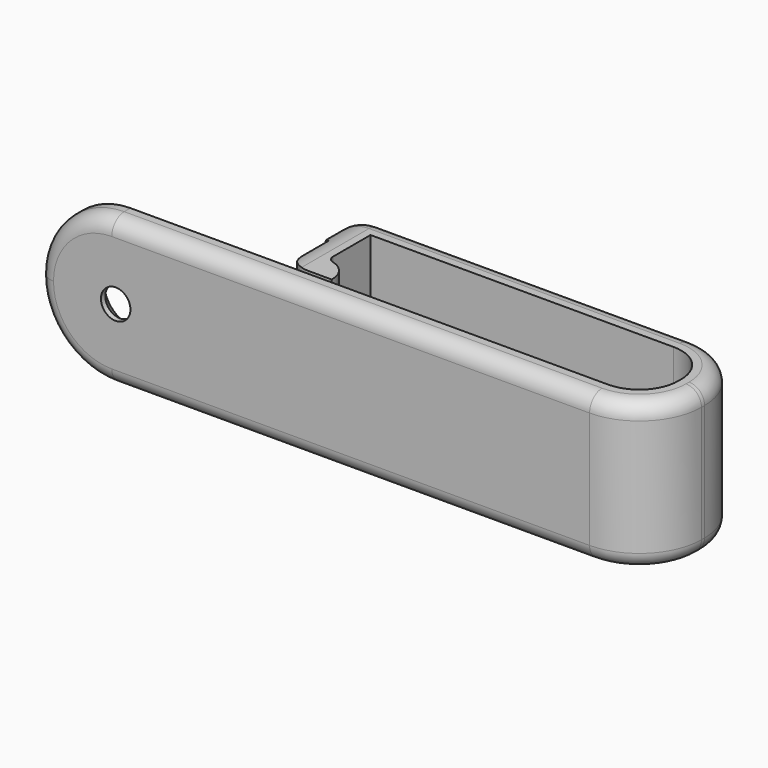
from build123d import *

# Parameters (mm, degrees)
F2_W            = 3
F2_H            = 3
F3_DEPTH        = 19
F5_R            = 9.49999
F6_R            = 5
F7_R            = 2
F8_R            = 1
F9_SIZE         = 2.99999
F10_D           = 3.7973
F10_CSINK_D     = 7.7978
F10_CSINK_ANGLE = 82
F11_R           = 2.9999


# Not quite as in the source:
# - a fillet or chamfer is up to 0.001 mm smaller than in the source, because OpenCascade refuses the exact size


with BuildPart() as f3:
    # F2 (on Top) → F3 (new body)
    with BuildSketch(Plane.XY):
        with BuildLine():
            Line((35.5, -27.8585158202), (-35.5, -27.8585158202))
            Line((-35.5, -27.8585158202), (-35.5, -30.8585158202))
            Line((-35.5, -30.8585158202), (35.5, -30.8585158202))
            ThreePointArc((35.5, -30.8585158202), (41.1568542495, -28.5153700696), (43.5, -22.8585158202))
            Line((43.5, -22.8585158202), (43.5, -22.3585158202))
            ThreePointArc((43.5, -22.3585158202), (41.1568542495, -16.7016615707), (35.5, -14.3585158202))
            Line((35.5, -14.3585158202), (-6.5, -14.3585158202))
            Line((-6.5, -14.3585158202), (-6.5, -16.3585158202))
            Line((-6.5, -16.3585158202), (-6.5, -17.3585158202))
            Line((-6.5, -17.3585158202), (-3.5, -17.3585158202))
            Line((-3.5, -17.3585158202), (35.5, -17.3585158202))
            ThreePointArc((35.5, -17.3585158202), (39.0355339059, -18.8229819142), (40.5, -22.3585158202))
            Line((40.5, -22.3585158202), (40.5, -22.8585158202))
            ThreePointArc((40.5, -22.8585158202), (39.0355339059, -26.3940497261), (35.5, -27.8585158202))
        make_face()
        with Locations((-2, -25.8585158202)):
            Rectangle(F2_W, F2_H)
        Polygon((-3.5, -24.3585158202), (-3.5, -17.3585158202), (-6.5, -17.3585158202), (-6.5, -27.3585158202), (-3.5, -27.3585158202), align=None)
        Polygon((-9.5, -17.3585158202), (-6.5, -17.3585158202), (-6.5, -16.3585158202), (-6.5, -14.3585158202), (-9.5, -14.3585158202), align=None)
    extrude(amount=F3_DEPTH)

    # F5 (radius 9.5 in the source; OpenCascade refuses exactly that, so slightly less here)
    f5_edges = [f3.edges().sort_by_distance(p)[0] for p in [
        (-35.5, -29.358516, 19),
        (-35.5, -29.358516, 0),
    ]]
    fillet(f5_edges, radius=F5_R)

    # F6
    f6_edges = [f3.edges().sort_by_distance(p)[0] for p in [
        (-9.5, -15.858516, 19),
        (-9.5, -15.858516, 0),
    ]]
    fillet(f6_edges, radius=F6_R)

    # F7
    f7_edges = [f3.edges().sort_by_distance(p)[0] for p in [
        (15.5, -14.358516, 0),
    ]]
    fillet(f7_edges, radius=F7_R)

    # F8
    f8_edges = [f3.edges().sort_by_distance(p)[0] for p in [
        (-3.5, -24.358516, 9.5),
    ]]
    fillet(f8_edges, radius=F8_R)

    # F9 (size 3 in the source; OpenCascade refuses exactly that, so slightly less here)
    f9_edges = [f3.edges().sort_by_distance(p)[0] for p in [
        (-6.5, -17.358516, 9.5),
    ]]
    chamfer(f9_edges, length=F9_SIZE)

    # F10 (through all)
    with Locations(Plane(origin=(0, -27.8585158202, 0), x_dir=(-1, 0, 0), z_dir=(0, 1, 0))):
        with Locations((25.5, 9.5)):
            CounterSinkHole(F10_D / 2, F10_CSINK_D / 2, counter_sink_angle=F10_CSINK_ANGLE)

    # F11 (radius 3 in the source; OpenCascade refuses exactly that, so slightly less here)
    f11_edges = [f3.edges().sort_by_distance(p)[0] for p in [
        (-0.5, -24.358516, 9.5),
        (-6.5, -27.358516, 9.5),
    ]]
    fillet(f11_edges, radius=F11_R)


solid = f3.part
